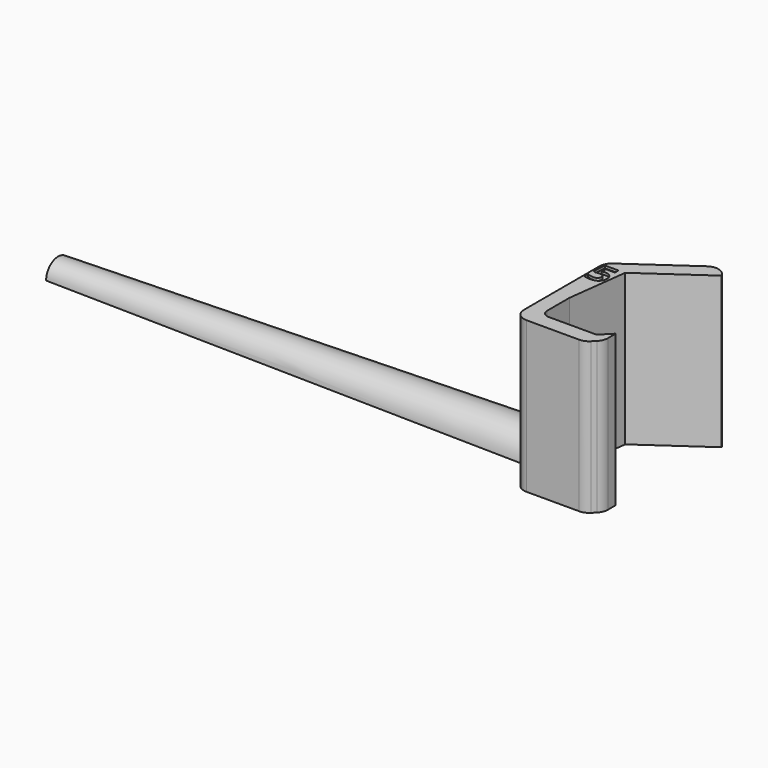
from build123d import *

# Parameters (mm, degrees)
F1_DEPTH      = 30
F2_TEXT_SIZE  = 6.9444444444
F3_DEPTH      = 0.5
F5_ANGLE_BACK = 90
F5_ANGLE      = 180


# Not quite as in the source:
# - Text() gives the source's letters only with a copy of the font that has no kerning and outlines rounded to 1/6400 em; it was checked with that copy


with BuildPart() as f1:
    # F0 (on Top) → F1 (new body)
    with BuildSketch(Plane.XY):
        with BuildLine():
            Line((16.1213203436, -6.7336657654), (14, -8.854986109))
            Line((14, -8.854986109), (4.5, -8.854986109))
            ThreePointArc((4.5, -8.854986109), (3.4393398282, -8.4156462808), (3, -7.354986109))
            Line((3, -7.354986109), (3, -1.854986109))
            Line((3, -1.854986109), (4.5, 10.145013891))
            Line((4.5, 10.145013891), (16.7872806643, 18.7486604363))
            Line((16.7872806643, 18.7486604363), (16.5004924462, 19.1582364584))
            ThreePointArc((16.5004924462, 19.1582364584), (14.8867327796, 20.1863147501), (13.0186712446, 19.7721754783))
            Line((13.0186712446, 19.7721754783), (1.0660589091, 11.4028662197))
            ThreePointArc((1.0660589091, 11.4028662197), (0.2824729171, 10.5093576421), (0, 9.354986109))
            Line((0, 9.354986109), (0, -9.354986109))
            ThreePointArc((0, -9.354986109), (0.732233047, -11.1227530619), (2.5, -11.854986109))
            Line((2.5, -11.854986109), (12.9644660941, -11.854986109))
            ThreePointArc((12.9644660941, -11.854986109), (13.921174675, -11.6646849403), (14.732233047, -11.1227530619))
            Line((14.732233047, -11.1227530619), (15.3890872965, -10.4658988125))
            ThreePointArc((15.3890872965, -10.4658988125), (15.9310191748, -9.6548404404), (16.1213203436, -8.6981318595))
            Line((16.1213203436, -8.6981318595), (16.1213203436, -6.7336657654))
        make_face()
    extrude(amount=F1_DEPTH)

    # F2 (on face) → F3 (cut)
    with BuildSketch(Plane.XY.offset(30)):
        with Locations((-0.1026475694, 5.145013891)):
            Text('5', F2_TEXT_SIZE, font='Open Sans', font_style=FontStyle.BOLD, text_align=(TextAlign.LEFT, TextAlign.BOTTOM))
    extrude(amount=-F3_DEPTH, mode=Mode.SUBTRACT)

    # F4 (on Front) → F5 (revolve)
    with BuildSketch(Plane.XZ, mode=Mode.PRIVATE) as f5_sk:
        Polygon((-100, 0), (0, 0), (0, 5), (-100, 3), align=None)
    revolve(f5_sk.sketch.rotate(Axis((-50, 0, 0), (-1, 0, 0)), -F5_ANGLE_BACK), axis=Axis((-50, 0, 0), (-1, 0, 0)), revolution_arc=F5_ANGLE)


solid = f1.part
